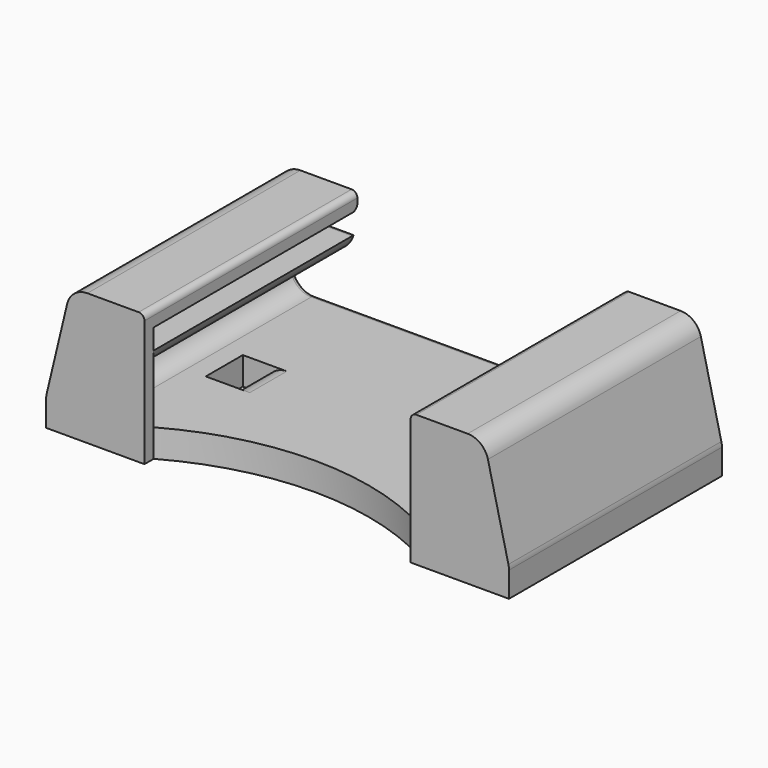
from build123d import *

# Parameters (mm, degrees)
F0_W        = 40
F0_H        = 23
F1_DEPTH    = 2.4
F2_W        = 8.5
F2_H        = 23
F3_DEPTH    = 9
F4_DEPTH    = 4
F5_W        = 4.35
F5_H        = 1.8
F5_W_2      = 5.3926127389
F5_H_2      = 4.4
F6_DEPTH    = 22
F7_DEPTH    = 23.001
F8_T1_DEPTH = 22
F8_T3_DEPTH = 24.0600856157
F8_T5_DEPTH = 30.1032426749
F8_T7_DEPTH = 4
F8_T9_DEPTH = 26.5
F9_R        = 0.5
F11_DEPTH   = 4.001


# Not quite as in the source:
# - a fillet or chamfer that OpenCascade refuses, or shapes differently, is made with other operations: its cross-section is extruded or revolved along the edge and cut away or added


with BuildPart() as f1:
    # F0 (on Top) → F1 (new body)
    with BuildSketch(Plane.XY):
        Rectangle(F0_W, F0_H)
        with BuildLine():
            ThreePointArc((-11.4, 1.5), (-9.4, -0.5), (-11.4, -2.5))
            Line((-11.4, -2.5), (-13.4, -2.5))
            Line((-13.4, -2.5), (-13.4, 1.5))
            Line((-13.4, 1.5), (-11.4, 1.5))
        make_face(mode=Mode.SUBTRACT)
        with BuildLine():
            ThreePointArc((11.4, -2.5), (9.4, -0.5), (11.4, 1.5))
            Line((11.4, 1.5), (13.4, 1.5))
            Line((13.4, 1.5), (13.4, -2.5))
            Line((13.4, -2.5), (11.4, -2.5))
        make_face(mode=Mode.SUBTRACT)
        with BuildLine():
            Line((-11.4, 1.5), (-11.4, -2.5))
            ThreePointArc((-11.4, -2.5), (-9.4, -0.5), (-11.4, 1.5))
        make_face()
        with BuildLine():
            Line((11.4, -2.5), (11.4, 1.5))
            ThreePointArc((11.4, 1.5), (9.4, -0.5), (11.4, -2.5))
        make_face()
    extrude(amount=-F1_DEPTH)

    # F2 (on face) → F3 (join)
    with BuildSketch(Plane.XY):
        with Locations((15.75, 0)):
            Rectangle(F2_W, F2_H)
        with Locations((-15.75, 0)):
            Rectangle(F2_W, F2_H)
    extrude(amount=F3_DEPTH)

    # F0 (on Top) → F4 (join)
    with BuildSketch(Plane.XY):
        with BuildLine():
            Line((-11.4, 1.5), (-11.4, -2.5))
            ThreePointArc((-11.4, -2.5), (-9.4, -0.5), (-11.4, 1.5))
        make_face()
        with BuildLine():
            Line((11.4, -2.5), (11.4, 1.5))
            ThreePointArc((11.4, 1.5), (9.4, -0.5), (11.4, -2.5))
        make_face()
    extrude(amount=-F4_DEPTH)

    # F5 (on face) → F6 (cut)
    with BuildSketch(Plane(origin=(0, 11.5, 0), x_dir=(-1, 0, 0), z_dir=(0, 1, 0))):
        with Locations((-13.675, 6.7)):
            Rectangle(F5_W, F5_H)
        with Locations((13.675, 6.7)):
            Rectangle(F5_W, F5_H)
        with Locations((14.1963063695, 2.2)):
            Rectangle(F5_W_2, F5_H_2)
        with Locations((-14.1963063695, 2.2)):
            Rectangle(F5_W_2, F5_H_2)
    extrude(amount=-F6_DEPTH, mode=Mode.SUBTRACT)

    # F5 (on face) → F7 (cut, through all)
    with BuildSketch(Plane(origin=(0, 11.5, 0), x_dir=(-1, 0, 0), z_dir=(0, 1, 0))):
        Polygon((-20, 0), (-17.85, 9), (-20, 9), align=None)
        Polygon((20, 9), (17.85, 9), (20, 0), align=None)
    extrude(amount=-F7_DEPTH, mode=Mode.SUBTRACT)

    # F8: fillet of radius 1.8 on 12 edges, made by hand

    # F8_s2 → F8_t1 (join)
    with BuildSketch(Plane.XZ.offset(-11.5)):
        with BuildLine():
            ThreePointArc((15.0926127389, 0), (16.3654049451, 0.5272077939), (16.8926127389, 1.8))
            Line((16.8926127389, 1.8), (16.8926127389, 0))
            Line((16.8926127389, 0), (15.0926127389, 0))
        make_face()
        with BuildLine():
            ThreePointArc((15.0926127389, 4.4), (16.3654049451, 3.8727922061), (16.8926127389, 2.6))
            Line((16.8926127389, 2.6), (16.8926127389, 4.4))
            Line((16.8926127389, 4.4), (15.0926127389, 4.4))
        make_face()
        with BuildLine():
            ThreePointArc((-16.8926127389, 2.6), (-16.3654049451, 3.8727922061), (-15.0926127389, 4.4))
            Line((-15.0926127389, 4.4), (-16.8926127389, 4.4))
            Line((-16.8926127389, 4.4), (-16.8926127389, 2.6))
        make_face()
        with BuildLine():
            ThreePointArc((-15.0926127389, 0), (-16.3654049451, 0.5272077939), (-16.8926127389, 1.8))
            Line((-16.8926127389, 1.8), (-16.8926127389, 0))
            Line((-16.8926127389, 0), (-15.0926127389, 0))
        make_face()
    extrude(amount=F8_T1_DEPTH)

    # F8_s4 → F8_t3 (cut)
    with BuildSketch(Plane.XZ.offset(-12.0300428079)):
        with BuildLine():
            ThreePointArc((20, -0.2120171231), (19.987641981, -0.0014556176), (19.9507376137, 0.2062146401))
            Line((19.9507376137, 0.2062146401), (20, 0))
            Line((20, 0), (20, -0.2120171231))
        make_face()
        with BuildLine():
            ThreePointArc((-20, -0.2120171231), (-19.987641981, -0.0014556176), (-19.9507376137, 0.2062146401))
            Line((-19.9507376137, 0.2062146401), (-20, 0))
            Line((-20, 0), (-20, -0.2120171231))
        make_face()
    extrude(amount=F8_T3_DEPTH, mode=Mode.SUBTRACT)

    # F8_s6 → F8_t5 (cut)
    with BuildSketch(Plane.XZ.offset(-15.0516213374)):
        with BuildLine():
            ThreePointArc((18.1800890788, 7.6182317633), (17.5445157637, 8.6129432356), (16.429351465, 9))
            Line((16.429351465, 9), (17.85, 9))
            Line((17.85, 9), (18.1800890788, 7.6182317633))
        make_face()
        with BuildLine():
            ThreePointArc((-18.1800890788, 7.6182317633), (-17.5445157637, 8.6129432356), (-16.429351465, 9))
            Line((-16.429351465, 9), (-17.85, 9))
            Line((-17.85, 9), (-18.1800890788, 7.6182317633))
        make_face()
    extrude(amount=F8_T5_DEPTH, mode=Mode.SUBTRACT)

    # F8_s8 → F8_t7 (cut)
    with BuildSketch(Plane.XZ.offset(-1.5)):
        with BuildLine():
            ThreePointArc((-9.6, 0), (-10.8727922061, -0.5272077939), (-11.4, -1.8))
            Line((-11.4, -1.8), (-11.4, 0))
            Line((-11.4, 0), (-9.6, 0))
        make_face()
        with BuildLine():
            ThreePointArc((9.6, 0), (10.8727922061, -0.5272077939), (11.4, -1.8))
            Line((11.4, -1.8), (11.4, 0))
            Line((11.4, 0), (9.6, 0))
        make_face()
    extrude(amount=F8_T7_DEPTH, mode=Mode.SUBTRACT)

    # F8_s10 → F8_t9 (cut)
    with BuildSketch(Plane.XZ.offset(-16)):
        with BuildLine():
            ThreePointArc((-11.5, 6.2), (-12.0272077939, 4.9272077939), (-13.3, 4.4))
            Line((-13.3, 4.4), (-11.5, 4.4))
            Line((-11.5, 4.4), (-11.5, 6.2))
        make_face()
        with BuildLine():
            ThreePointArc((11.5, 6.2), (12.0272077939, 4.9272077939), (13.3, 4.4))
            Line((13.3, 4.4), (11.5, 4.4))
            Line((11.5, 4.4), (11.5, 6.2))
        make_face()
    extrude(amount=F8_T9_DEPTH, mode=Mode.SUBTRACT)

    # F9
    f9_edges = [f1.edges().sort_by_distance(p)[0] for p in [
        (-15.85, 11.5, 6.7),
        (-13.675, 11.5, 7.6),
        (-13.697504, 11.5, 5.8),
        (13.697504, 11.5, 5.8),
        (13.675, 11.5, 7.6),
        (15.85, 11.5, 6.7),
        (11.5, 0, 9),
        (-11.5, 0, 9),
        (0, 11.5, 0),
        (12.177503, 11.5, 4.792875),
        (14.196306, 11.5, 4.4),
        (16.365405, 11.5, 3.872792),
        (16.892613, 11.5, 2.2),
        (16.365405, 11.5, 0.527208),
        (-16.365405, 11.5, 0.527208),
        (-16.892613, 11.5, 2.2),
        (-16.365405, 11.5, 3.872792),
        (-14.196306, 11.5, 4.4),
        (-12.177503, 11.5, 4.792875),
    ]]
    fillet(f9_edges, radius=F9_R)

    # F10 (on face) → F11 (cut, through all)
    with BuildSketch(Plane.XY):
        with BuildLine():
            Line((11.5, -11.5), (11.5, -10.5))
            ThreePointArc((11.5, -10.5), (0, -7.5), (-11.5, -10.5))
            Line((-11.5, -10.5), (-11.5, -11.5))
            Line((-11.5, -11.5), (11.5, -11.5))
        make_face()
    extrude(amount=-F11_DEPTH, mode=Mode.SUBTRACT)


solid = f1.part
